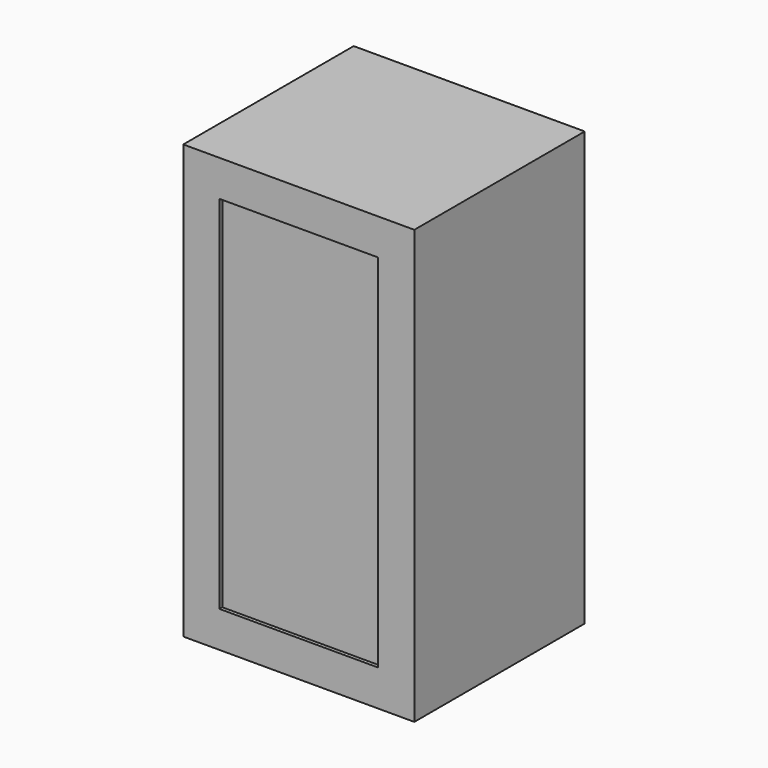
from build123d import *

# Parameters (mm, degrees)
F0_W     = 279.4
F0_H     = 635
F1_DEPTH = 374.65
F2_DEPTH = 6.35


# Not quite as in the source:
# - a feature names something its author has since deleted; it is built from what else it names


with BuildPart() as f1:
    # F0 (on Front) → F1 (new body)
    with BuildSketch(Plane.XZ):
        Polygon((263.9267770052, 0), (289.3267770052, 0), (289.3267770052, 762), (263.9267770052, 762), (-117.0732229948, 762), (-117.0732229948, 0), align=None)
        with Locations((86.1267770052, 381)):
            Rectangle(F0_W, F0_H, mode=Mode.SUBTRACT)
        with Locations((86.1267770052, 381)):
            Rectangle(F0_W, F0_H)
    extrude(amount=-F1_DEPTH)

    # F0 (on Front) → F2 (cut)
    with BuildSketch(Plane.XZ):
        with Locations((86.1267770052, 381)):
            Rectangle(F0_W, F0_H)
    extrude(amount=-F2_DEPTH, mode=Mode.SUBTRACT)


solid = f1.part
